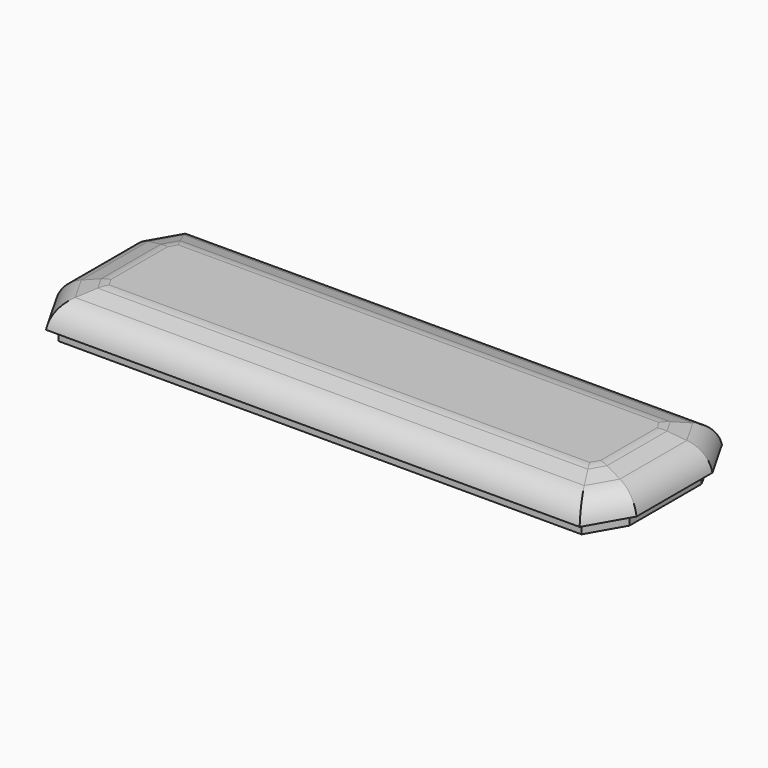
from build123d import *

# Parameters (mm, degrees)
F0_W         = 90
F0_H         = 30
F1_DEPTH     = 5
F2_W         = 1
F2_H         = 2
F4_SIZE2     = 2
F4_SIZE      = 7
F5_T1_DEPTH  = 121.5034235835
F5_T3_DEPTH  = 85.3768581194
F5_T5_DEPTH  = 51.611107996
F5_T7_DEPTH  = 15.783471497
F5_T9_DEPTH  = 71.594276912
F5_T11_DEPTH = 5.6424225565
F5_T13_DEPTH = 51.611107996
F5_T15_DEPTH = 5.6424225565
F5_T17_DEPTH = 51.611107996
F5_T19_DEPTH = 5.6424225565
F5_T21_DEPTH = 5.6424225565
F5_T23_DEPTH = 51.611107996


# Not quite as in the source:
# - a fillet or chamfer that OpenCascade refuses, or shapes differently, is made with other operations: its cross-section is extruded or revolved along the edge and cut away or added


with BuildPart() as f1:
    # F0 (on Top) → F1 (new body)
    with BuildSketch(Plane.XY):
        Polygon((-45, -15), (-45, 15), (-49, 8), (-49, -8), align=None)
        Polygon((49, 8), (45, 15), (45, -15), (49, -8), align=None)
        Rectangle(F0_W, F0_H)
    extrude(amount=F1_DEPTH)

    # F3: sweep along a path in F3_path
    with BuildLine(Plane(origin=(45, -15, 0), x_dir=(0, -1, 0), z_dir=(0, 0, -1))) as f3_path:
        Line((0, 0), (0, 90))
        Line((0, 90), (-7, 94))
        Line((-7, 94), (-23, 94))
        Line((-23, 94), (-30, 90))
        Line((-30, 90), (-30, 0))
        Line((-30, 0), (-23, -4))
        Line((-23, -4), (-7, -4))
        Line((-7, -4), (0, 0))
    # F2 (on Right) → F3 (sweep)
    with BuildSketch(Plane.YZ):
        with Locations((-13, -1)):
            Rectangle(F2_W, F2_H)
    sweep(path=f3_path.line, transition=Transition.RIGHT)

    # F4
    f4_edges = [f1.edges().sort_by_distance(p)[0] for p in [
        (-49, 0, 5),
        (-47, -11.5, 5),
        (-47, 11.5, 5),
        (47, -11.5, 5),
        (49, 0, 5),
        (47, 11.5, 5),
        (0, -15, 5),
        (0, 15, 5),
    ]]
    f4_side = f1.faces().sort_by_distance((0, 0, 5))[0]
    chamfer(f4_edges, length=F4_SIZE, length2=F4_SIZE2, reference=f4_side)

    # F5: fillet of radius 5 on 16 edges, made by hand

    # F5_s2 → F5_t1 (cut)
    with BuildSketch(Plane.YZ.offset(-60.7517117917)):
        with BuildLine():
            ThreePointArc((15, 0), (13.8034764966, 2.5282074371), (11.4363180932, 4.0181948305))
            Line((11.4363180932, 4.0181948305), (15, 3))
            Line((15, 3), (15, 0))
        make_face()
        with BuildLine():
            ThreePointArc((-15, 0), (-13.8034764966, 2.5282074371), (-11.4363180932, 4.0181948305))
            Line((-11.4363180932, 4.0181948305), (-15, 3))
            Line((-15, 3), (-15, 0))
        make_face()
    extrude(amount=F5_T1_DEPTH, mode=Mode.SUBTRACT)

    # F5_s4 → F5_t3 (cut)
    with BuildSketch(Plane.YZ.offset(-42.6884290597)):
        with BuildLine():
            ThreePointArc((8.6733309163, 4.8076197382), (7.9932313362, 4.9516713689), (7.2997252768, 5))
            Line((7.2997252768, 5), (8, 5))
            Line((8, 5), (8.6733309163, 4.8076197382))
        make_face()
        with BuildLine():
            ThreePointArc((-7.2997252768, 5), (-7.9932313362, 4.9516713689), (-8.6733309163, 4.8076197382))
            Line((-8.6733309163, 4.8076197382), (-8, 5))
            Line((-8, 5), (-7.2997252768, 5))
        make_face()
    extrude(amount=F5_T3_DEPTH, mode=Mode.SUBTRACT)

    # F5_s6 → F5_t5 (cut)
    with BuildSketch(Plane(origin=(-22.4066273783, 39.211597912, 0), x_dir=(0, 0, 1), z_dir=(0.4961389384, -0.8682431421, 0))):
        with BuildLine():
            ThreePointArc((0, 46.513025471), (2.5282074371, 45.3165019675), (4.0181948305, 42.9493435641))
            Line((4.0181948305, 42.9493435641), (3, 46.513025471))
            Line((3, 46.513025471), (0, 46.513025471))
        make_face()
    extrude(amount=F5_T5_DEPTH, mode=Mode.SUBTRACT)

    # F5_s8 → F5_t7 (cut)
    with BuildSketch(Plane.XZ.offset(-7.8917357485)):
        with BuildLine():
            ThreePointArc((-41.2997252768, 5), (-41.9932313362, 4.9516713689), (-42.6733309163, 4.8076197382))
            Line((-42.6733309163, 4.8076197382), (-42, 5))
            Line((-42, 5), (-41.2997252768, 5))
        make_face()
        with BuildLine():
            ThreePointArc((41.2997252768, 5), (41.9932313362, 4.9516713689), (42.6733309163, 4.8076197382))
            Line((42.6733309163, 4.8076197382), (42, 5))
            Line((42, 5), (41.2997252768, 5))
        make_face()
    extrude(amount=F5_T7_DEPTH, mode=Mode.SUBTRACT)

    # F5_s10 → F5_t9 (cut)
    with BuildSketch(Plane.XZ.offset(-35.797138456)):
        with BuildLine():
            ThreePointArc((-49, 0), (-47.8034764966, 2.5282074371), (-45.4363180932, 4.0181948305))
            Line((-45.4363180932, 4.0181948305), (-49, 3))
            Line((-49, 3), (-49, 0))
        make_face()
        with BuildLine():
            ThreePointArc((49, 0), (47.8034764966, 2.5282074371), (45.4363180932, 4.0181948305))
            Line((45.4363180932, 4.0181948305), (49, 3))
            Line((49, 3), (49, 0))
        make_face()
    extrude(amount=F5_T9_DEPTH, mode=Mode.SUBTRACT)

    # F5_s12 → F5_t11 (cut)
    with BuildSketch(Plane(origin=(-8.5616705046, 14.982923383, 0), x_dir=(0, 0, 1), z_dir=(0.4961389384, -0.8682431421, 0))):
        with BuildLine():
            ThreePointArc((5, 38.8127507478), (4.9516713689, 39.5062568072), (4.8076197382, 40.1863563872))
            Line((4.8076197382, 40.1863563872), (5, 39.513025471))
            Line((5, 39.513025471), (5, 38.8127507478))
        make_face()
    extrude(amount=F5_T11_DEPTH, mode=Mode.SUBTRACT)

    # F5_s14 → F5_t13 (cut)
    with BuildSketch(Plane(origin=(3.1996529503, 5.599392663, 0), x_dir=(0, 0, 1), z_dir=(-0.4961389384, -0.8682431421, 0))):
        with BuildLine():
            ThreePointArc((0, 46.513025471), (2.5282074371, 45.3165019675), (4.0181948305, 42.9493435641))
            Line((4.0181948305, 42.9493435641), (3, 46.513025471))
            Line((3, 46.513025471), (0, 46.513025471))
        make_face()
    extrude(amount=F5_T13_DEPTH, mode=Mode.SUBTRACT)

    # F5_s16 → F5_t15 (cut)
    with BuildSketch(Plane(origin=(-5.7622449676, -10.0839286934, 0), x_dir=(0, 0, 1), z_dir=(-0.4961389384, -0.8682431421, 0))):
        with BuildLine():
            ThreePointArc((4.8076197382, 40.1863563872), (4.9516713689, 39.5062568072), (5, 38.8127507478))
            Line((5, 38.8127507478), (5, 39.513025471))
            Line((5, 39.513025471), (4.8076197382, 40.1863563872))
        make_face()
    extrude(amount=F5_T15_DEPTH, mode=Mode.SUBTRACT)

    # F5_s18 → F5_t17 (cut)
    with BuildSketch(Plane(origin=(22.4066273783, -39.211597912, 0), x_dir=(0, 0, 1), z_dir=(-0.4961389384, 0.8682431421, 0))):
        with BuildLine():
            ThreePointArc((0, 46.513025471), (2.5282074371, 45.3165019675), (4.0181948305, 42.9493435641))
            Line((4.0181948305, 42.9493435641), (3, 46.513025471))
            Line((3, 46.513025471), (0, 46.513025471))
        make_face()
    extrude(amount=F5_T17_DEPTH, mode=Mode.SUBTRACT)

    # F5_s20 → F5_t19 (cut)
    with BuildSketch(Plane(origin=(8.5616705046, -14.982923383, 0), x_dir=(0, 0, 1), z_dir=(-0.4961389384, 0.8682431421, 0))):
        with BuildLine():
            ThreePointArc((5, 38.8127507478), (4.9516713689, 39.5062568072), (4.8076197382, 40.1863563872))
            Line((4.8076197382, 40.1863563872), (5, 39.513025471))
            Line((5, 39.513025471), (5, 38.8127507478))
        make_face()
    extrude(amount=F5_T19_DEPTH, mode=Mode.SUBTRACT)

    # F5_s22 → F5_t21 (cut)
    with BuildSketch(Plane(origin=(5.7622449676, 10.0839286934, 0), x_dir=(0, 0, 1), z_dir=(0.4961389384, 0.8682431421, 0))):
        with BuildLine():
            ThreePointArc((5, 38.8127507478), (4.9516713689, 39.5062568072), (4.8076197382, 40.1863563872))
            Line((4.8076197382, 40.1863563872), (5, 39.513025471))
            Line((5, 39.513025471), (5, 38.8127507478))
        make_face()
    extrude(amount=F5_T21_DEPTH, mode=Mode.SUBTRACT)

    # F5_s24 → F5_t23 (cut)
    with BuildSketch(Plane(origin=(-3.1996529503, -5.599392663, 0), x_dir=(0, 0, 1), z_dir=(0.4961389384, 0.8682431421, 0))):
        with BuildLine():
            ThreePointArc((0, 46.513025471), (2.5282074371, 45.3165019675), (4.0181948305, 42.9493435641))
            Line((4.0181948305, 42.9493435641), (3, 46.513025471))
            Line((3, 46.513025471), (0, 46.513025471))
        make_face()
    extrude(amount=F5_T23_DEPTH, mode=Mode.SUBTRACT)


solid = f1.part
